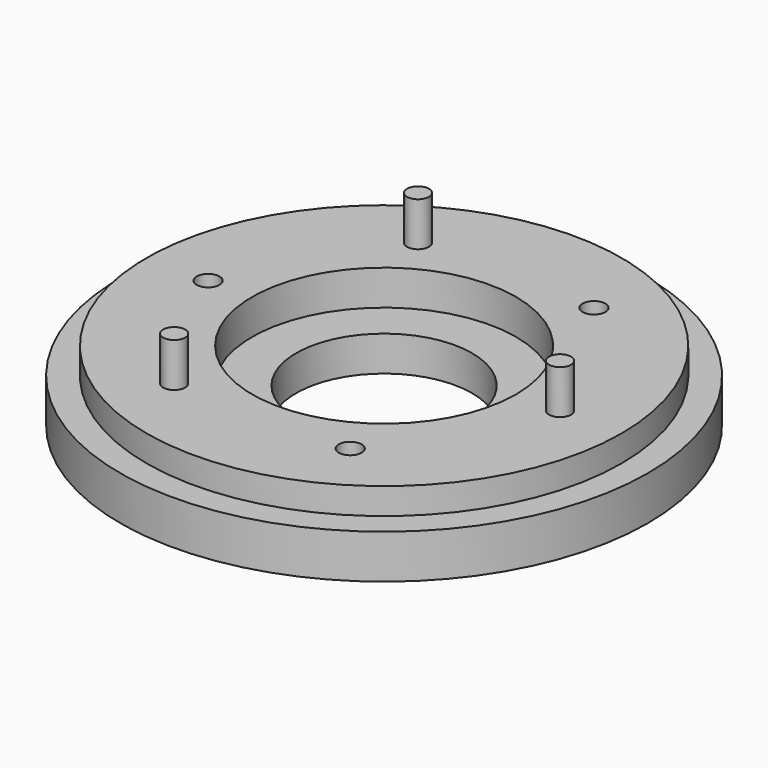
from build123d import *

# Parameters (mm, degrees)
F2_R            = 1.25
F3_DEPTH        = 5
F3_COPIES_COUNT = 3
F5_D            = 2.6
F5_CBORE_D      = 5
F5_CBORE_DEPTH  = 4
F5_COPIES_COUNT = 3
F6_W            = 3
F6_H            = 3


# Not quite as in the source:
# - a pattern or mirror of a feature is missing from the dataset's text; its kind, count and spacing are read off the source's solid


with BuildPart() as f1:
    # F0 (on Front) → F1 (revolve)
    with BuildSketch(Plane.XZ):
        Polygon((10, 4), (10, 0), (30, 0), (30, 8), (15, 8), (15, 4), align=None)
    revolve(axis=Axis((0, 0, 1.9594207406), (0, 0, -1)))

    # F2 (on face) → F3 (join)
    with BuildSketch(Plane.XY.offset(8)):
        with Locations((20, 0)):
            Circle(F2_R)
    f3 = extrude(amount=F3_DEPTH)

    # F3_copies: F3 ×3 about axis
    f3_copies_axis = Axis((0, 0, 0), (0, 0, 1))
    for i in range(1, F3_COPIES_COUNT):
        add(f3.rotate(f3_copies_axis, i * 360 / F3_COPIES_COUNT))

    # F5 (through all)
    with Locations(Plane(origin=(0, 0, 0), x_dir=(1, 0, 0), z_dir=(0, 0, -1))):
        with Locations((-20, 0)):
            f5 = CounterBoreHole(F5_D / 2, F5_CBORE_D / 2, F5_CBORE_DEPTH)

    # F5_copies: F5 ×3 about axis
    f5_copies_axis = Axis((0, 0, 0), (0, 0, 1))
    for i in range(1, F5_COPIES_COUNT):
        add(f5.rotate(f5_copies_axis, i * 360 / F5_COPIES_COUNT), mode=Mode.SUBTRACT)

    # F6 (on Front) → F7 (revolve, cut)
    with BuildSketch(Plane.XZ):
        with Locations((28.5, 6.5)):
            Rectangle(F6_W, F6_H)
    revolve(axis=Axis((0, 0, 1.9594207406), (0, 0, -1)), mode=Mode.SUBTRACT)


solid = f1.part
